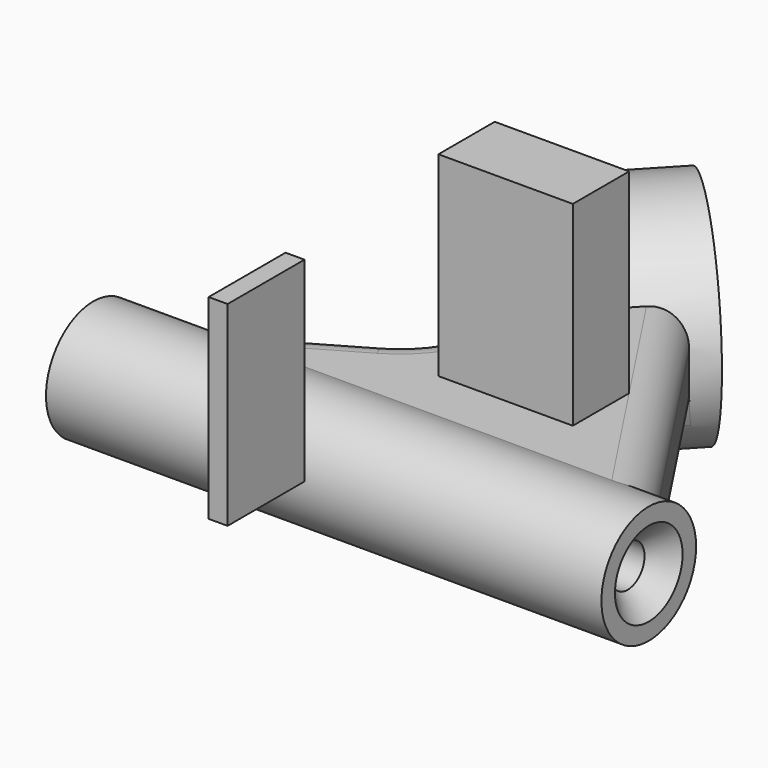
from build123d import *

# Parameters (mm, degrees)
F1_DEPTH      = 12.7
F3_R          = 13.9527302744
F4_DEPTH      = 39.2973385505
F5_R          = 14
F6_DEPTH      = 131.4124912024
F7_R          = 5
F8_DEPTH      = 131.4134912024
F9_T2_ANGLE   = 90
F9_T4_ANGLE   = 90
F9_T6_ANGLE   = 180
F10_T4_DEPTH  = 117.0418308162
F10_S5_R      = 14
F10_T6_DEPTH  = 64
F10_S7_R      = 26.0617093966
F10_T8_DEPTH  = 64
F10_T12_ANGLE = 141.4711994172
F10_S13_R     = 26.0617093966
F10_T14_DEPTH = 40
F10_T18_ANGLE = 141.4711994172
F10_T23_DEPTH = 117.0418308162
F10_S24_R     = 14
F10_T25_DEPTH = 64
F10_S26_R     = 26.0617093966
F10_T27_DEPTH = 64
F10_T31_ANGLE = 141.4711994172
F10_S32_R     = 26.0617093966
F10_T33_DEPTH = 40
F10_T37_ANGLE = 141.4711994172
F10_T42_DEPTH = 99.0169613427
F10_S43_R     = 14
F10_T44_DEPTH = 55
F10_T48_DEPTH = 99.0169613427
F10_S49_R     = 14
F10_T50_DEPTH = 55
F11_W         = 31.7987574321
F11_H         = 16.6520640796
F12_DEPTH     = 46.2048202753
F11_W_2       = 4.480779171
F11_H_2       = 22.7374769747


# Not quite as in the source:
# - a fillet or chamfer that OpenCascade refuses, or shapes differently, is made with other operations: its cross-section is extruded or revolved along the edge and cut away or added


with BuildPart() as f1:
    # F0 (on Top) → F1 (new body, symmetric)
    with BuildSketch(Plane.XY):
        with BuildLine():
            Line((-127, 0), (0, 0))
            Line((0, 0), (-59.1591745615, 89.741513133))
            Line((-59.1591745615, 89.741513133), (-86.0974043608, 61.1301064491))
            ThreePointArc((-86.0974043608, 61.1301064491), (-73.1823881205, 44.2487624745), (-83.0059094878, 25.4))
            Line((-83.0059094878, 25.4), (-127, 0))
        make_face()
    extrude(amount=F1_DEPTH, both=True)

    # F0 (on Top) → F2 (revolve)
    with BuildSketch(Plane.XY):
        Polygon((-86.0974043608, 61.1301064491), (-59.1591745615, 89.741513133), (-78.134051587, 107.6067514057), (-105.0722813863, 78.9953447218), align=None)
    revolve(axis=Axis((-72.6282894611, 75.4358097911, 0), (0.6854975628, 0.7280749216, 0)))

    # F3 (on face) → F4 (cut, through all)
    with BuildSketch(Plane(origin=(16.9901086158, 18.0453916546, 0), x_dir=(-0.7280749216, 0.6854975628, 0), z_dir=(0.6854975628, 0.7280749216, 0))):
        with Locations((104.5898999113, 0)):
            Circle(F3_R)
    extrude(amount=-F4_DEPTH, mode=Mode.SUBTRACT)

    # F5 (on Right) → F6 (join)
    with BuildSketch(Plane.YZ):
        Circle(F5_R)
    extrude(amount=-F6_DEPTH)

    # F7 (on face) → F8 (cut, through all)
    with BuildSketch(Plane.YZ):
        Circle(F7_R)
    extrude(amount=-F8_DEPTH, mode=Mode.SUBTRACT)

    # F9: chamfer of 5 on 4 edges, made by hand

    # F9_s1 → F9_t2 (revolve, cut)
    with BuildSketch(Plane.XZ):
        Polygon((0, -10), (-5, -5), (0, -5), align=None)
    revolve(axis=Axis((0, 0, 0), (1, 0, 0)), revolution_arc=F9_T2_ANGLE, mode=Mode.SUBTRACT)

    # F9_s3 → F9_t4 (revolve, cut)
    with BuildSketch(Plane.XY):
        Polygon((0, 10), (-5, 5), (0, 5), align=None)
    revolve(axis=Axis((0, 0, 0), (1, 0, 0)), revolution_arc=F9_T4_ANGLE, mode=Mode.SUBTRACT)

    # F9_s5 → F9_t6 (revolve, cut)
    with BuildSketch(Plane.XZ):
        Polygon((0, 10), (-5, 5), (0, 5), align=None)
    revolve(axis=Axis((0, 0, 0), (1, 0, 0)), revolution_arc=F9_T6_ANGLE, mode=Mode.SUBTRACT)

    # F9_s7 → F9_t8 (revolve, cut)
    with BuildSketch(Plane.XY):
        Polygon((-131.4124912024, 10), (-126.4124912024, 5), (-131.4124912024, 5), align=None)
    revolve(axis=Axis((-131.4124912024, 0, 0), (1, 0, 0)), mode=Mode.SUBTRACT)

    # F10: fillet of radius 8 on 6 edges, made by hand


with BuildPart() as f10_tool2:
    # F10_s3 → F10_t4 (new body)
    with BuildSketch(Plane(origin=(7.123948143, -10.8066735308, 0), x_dir=(0, 0, 1), z_dir=(-0.5503870348, 0.834909643, 0))):
        with BuildLine():
            ThreePointArc((12.7, -8), (10.3568542495, -2.3431457505), (4.7, 0))
            Line((4.7, 0), (12.7, 0))
            Line((12.7, 0), (12.7, -8))
        make_face()
    extrude(amount=F10_T4_DEPTH)

    # F10_s5 → F10_t6 (cut, symmetric)
    with BuildSketch(Plane.YZ.offset(-28.4)):
        Circle(F10_S5_R)
    extrude(amount=F10_T6_DEPTH, both=True, mode=Mode.SUBTRACT)

    # F10_s7 → F10_t8 (cut, symmetric)
    with BuildSketch(Plane(origin=(4.5242839142, 4.8052944825, 0), x_dir=(0, 0, 1), z_dir=(-0.6854975628, -0.7280749216, 0))):
        with Locations((0, 104.5898999113)):
            Circle(F10_S7_R)
    extrude(amount=F10_T8_DEPTH, both=True, mode=Mode.SUBTRACT)


with BuildPart() as f1_1:
    add(f1.part)

    # F10_t1: cut F10_tool2
    add(f10_tool2.part, mode=Mode.SUBTRACT)


with BuildPart() as f10_tool10:
    # F10_s11 → F10_t12 (revolve)
    with BuildSketch(Plane(origin=(-97.0992752721, 14.5614862447, 0), x_dir=(0, 0, 1), z_dir=(-0.9889414398, 0.1483065361, 0))):
        with BuildLine():
            ThreePointArc((-4.7, 48.0882621603), (-10.3568542495, 50.4314079108), (-12.7, 56.0882621603))
            Line((-12.7, 56.0882621603), (-12.7, 48.0882621603))
            Line((-12.7, 48.0882621603), (-4.7, 48.0882621603))
        make_face()
    revolve(axis=Axis((-92.9031110442, 42.5424559485, -12.7), (0, 0, -1)), revolution_arc=F10_T12_ANGLE)

    # F10_s13 → F10_t14 (cut, symmetric)
    with BuildSketch(Plane(origin=(-12.2018566171, -12.9597336043, 0), x_dir=(0, 0, 1), z_dir=(-0.6854975628, -0.7280749216, 0))):
        with Locations((0, 104.5898999113)):
            Circle(F10_S13_R)
    extrude(amount=F10_T14_DEPTH, both=True, mode=Mode.SUBTRACT)


with BuildPart() as f1_2:
    add(f1_1.part)

    # F10_t9: cut F10_tool10
    add(f10_tool10.part, mode=Mode.SUBTRACT)


with BuildPart() as f10_tool16:
    # F10_s17 → F10_t18 (revolve)
    with BuildSketch(Plane(origin=(-97.0992752721, 14.5614862447, 0), x_dir=(0, 0, 1), z_dir=(-0.9889414398, 0.1483065361, 0))):
        with BuildLine():
            ThreePointArc((-4.7, 48.0882621603), (-10.3568542495, 50.4314079108), (-12.7, 56.0882621603))
            Line((-12.7, 56.0882621603), (-12.7, 48.0882621603))
            Line((-12.7, 48.0882621603), (-4.7, 48.0882621603))
        make_face()
    revolve(axis=Axis((-92.9031110442, 42.5424559485, -12.7), (0, 0, -1)), revolution_arc=F10_T18_ANGLE)

    split(bisect_by=Plane(origin=(-9.9481211835, -10.5660150293, 0), x_dir=(0, 0, 1), z_dir=(-0.6854975628, -0.7280749216, 0)), keep=Keep.TOP)


with BuildPart() as f1_3:
    add(f1_2.part)

    # F10_t15: cut F10_tool16
    add(f10_tool16.part, mode=Mode.SUBTRACT)


with BuildPart() as f10_tool21:
    # F10_s22 → F10_t23 (new body)
    with BuildSketch(Plane(origin=(7.123948143, -10.8066735308, 0), x_dir=(0, 0, 1), z_dir=(-0.5503870348, 0.834909643, 0))):
        with BuildLine():
            ThreePointArc((-12.7, -8), (-10.3568542495, -2.3431457505), (-4.7, 0))
            Line((-4.7, 0), (-12.7, 0))
            Line((-12.7, 0), (-12.7, -8))
        make_face()
    extrude(amount=F10_T23_DEPTH)

    # F10_s24 → F10_t25 (cut, symmetric)
    with BuildSketch(Plane.YZ.offset(-28.4)):
        Circle(F10_S24_R)
    extrude(amount=F10_T25_DEPTH, both=True, mode=Mode.SUBTRACT)

    # F10_s26 → F10_t27 (cut, symmetric)
    with BuildSketch(Plane(origin=(4.5242839142, 4.8052944825, 0), x_dir=(0, 0, 1), z_dir=(-0.6854975628, -0.7280749216, 0))):
        with Locations((0, 104.5898999113)):
            Circle(F10_S26_R)
    extrude(amount=F10_T27_DEPTH, both=True, mode=Mode.SUBTRACT)


with BuildPart() as f1_4:
    add(f1_3.part)

    # F10_t20: cut F10_tool21
    add(f10_tool21.part, mode=Mode.SUBTRACT)


with BuildPart() as f10_tool29:
    # F10_s30 → F10_t31 (revolve)
    with BuildSketch(Plane(origin=(-97.0992752721, 14.5614862447, 0), x_dir=(0, 0, 1), z_dir=(-0.9889414398, 0.1483065361, 0))):
        with BuildLine():
            ThreePointArc((4.7, 48.0882621603), (10.3568542495, 50.4314079108), (12.7, 56.0882621603))
            Line((12.7, 56.0882621603), (12.7, 48.0882621603))
            Line((12.7, 48.0882621603), (4.7, 48.0882621603))
        make_face()
    revolve(axis=Axis((-92.9031110442, 42.5424559485, 12.7), (0, 0, -1)), revolution_arc=F10_T31_ANGLE)

    # F10_s32 → F10_t33 (cut, symmetric)
    with BuildSketch(Plane(origin=(-12.2018566171, -12.9597336043, 0), x_dir=(0, 0, 1), z_dir=(-0.6854975628, -0.7280749216, 0))):
        with Locations((0, 104.5898999113)):
            Circle(F10_S32_R)
    extrude(amount=F10_T33_DEPTH, both=True, mode=Mode.SUBTRACT)


with BuildPart() as f1_5:
    add(f1_4.part)

    # F10_t28: cut F10_tool29
    add(f10_tool29.part, mode=Mode.SUBTRACT)


with BuildPart() as f10_tool35:
    # F10_s36 → F10_t37 (revolve)
    with BuildSketch(Plane(origin=(-97.0992752721, 14.5614862447, 0), x_dir=(0, 0, 1), z_dir=(-0.9889414398, 0.1483065361, 0))):
        with BuildLine():
            ThreePointArc((4.7, 48.0882621603), (10.3568542495, 50.4314079108), (12.7, 56.0882621603))
            Line((12.7, 56.0882621603), (12.7, 48.0882621603))
            Line((12.7, 48.0882621603), (4.7, 48.0882621603))
        make_face()
    revolve(axis=Axis((-92.9031110442, 42.5424559485, 12.7), (0, 0, -1)), revolution_arc=F10_T37_ANGLE)

    split(bisect_by=Plane(origin=(-9.9481211835, -10.5660150293, 0), x_dir=(0, 0, 1), z_dir=(-0.6854975628, -0.7280749216, 0)), keep=Keep.TOP)


with BuildPart() as f1_6:
    add(f1_5.part)

    # F10_t34: cut F10_tool35
    add(f10_tool35.part, mode=Mode.SUBTRACT)


with BuildPart() as f10_tool40:
    # F10_s41 → F10_t42 (new body)
    with BuildSketch(Plane(origin=(-51.2559094878, -29.5926131403, 0), x_dir=(0, 0, 1), z_dir=(-0.8660254038, -0.5, 0))):
        with BuildLine():
            ThreePointArc((4.7, 63.5), (10.3568542495, 61.1568542495), (12.7, 55.5))
            Line((12.7, 55.5), (12.7, 63.5))
            Line((12.7, 63.5), (4.7, 63.5))
        make_face()
    extrude(amount=F10_T42_DEPTH)

    # F10_s43 → F10_t44 (cut, symmetric)
    with BuildSketch(Plane.YZ.offset(-123.9)):
        Circle(F10_S43_R)
    extrude(amount=F10_T44_DEPTH, both=True, mode=Mode.SUBTRACT)


with BuildPart() as f1_7:
    add(f1_6.part)

    # F10_t39: cut F10_tool40
    add(f10_tool40.part, mode=Mode.SUBTRACT)


with BuildPart() as f10_tool46:
    # F10_s47 → F10_t48 (new body)
    with BuildSketch(Plane(origin=(-51.2559094878, -29.5926131403, 0), x_dir=(0, 0, 1), z_dir=(-0.8660254038, -0.5, 0))):
        with BuildLine():
            ThreePointArc((-4.7, 63.5), (-10.3568542495, 61.1568542495), (-12.7, 55.5))
            Line((-12.7, 55.5), (-12.7, 63.5))
            Line((-12.7, 63.5), (-4.7, 63.5))
        make_face()
    extrude(amount=F10_T48_DEPTH)

    # F10_s49 → F10_t50 (cut, symmetric)
    with BuildSketch(Plane.YZ.offset(-123.9)):
        Circle(F10_S49_R)
    extrude(amount=F10_T50_DEPTH, both=True, mode=Mode.SUBTRACT)


with BuildPart() as f1_8:
    add(f1_7.part)

    # F10_t45: cut F10_tool46
    add(f10_tool46.part, mode=Mode.SUBTRACT)

    # F11 (on face) → F12 (join)
    with BuildSketch(Plane.XY.offset(12.7)):
        with Locations((-48.593450428, 26.7340157452)):
            Rectangle(F11_W, F11_H)
    extrude(amount=F12_DEPTH)


with BuildPart() as f12:
    # F11 (on face) → F12, piece 2 (new body)
    with BuildSketch(Plane.XY.offset(12.7)):
        with Locations((-59.7145333886, -41.3479376584)):
            Rectangle(F11_W_2, F11_H_2)
    extrude(amount=F12_DEPTH)


solid = Compound([f1_8.part, f12.part])
